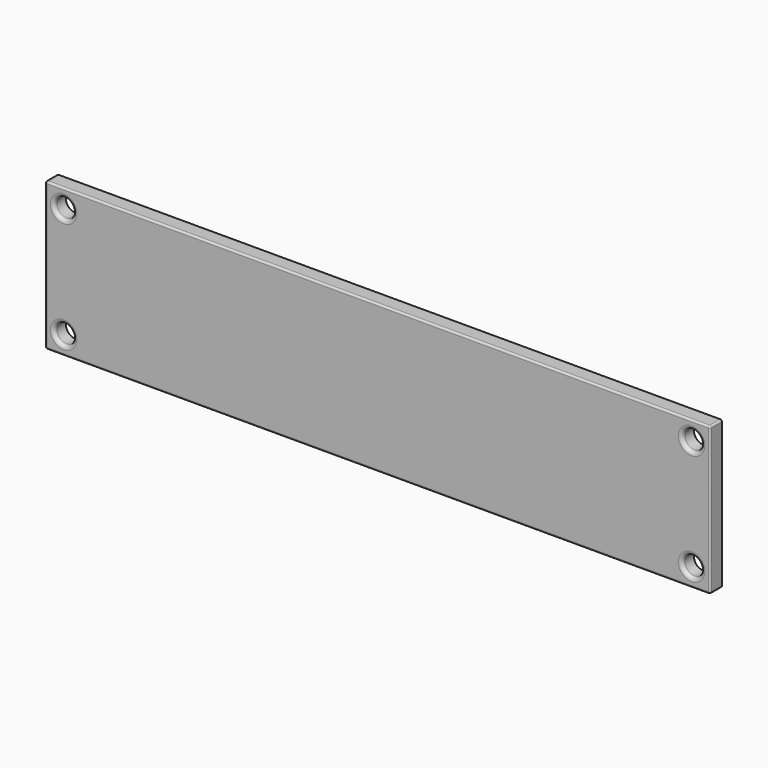
from build123d import *

# Parameters (mm, degrees)
F0_W         = 180
F0_H         = 40
F0_R         = 2.5751263091
F1_DEPTH     = 4
F2_R         = 1
F3_R         = 0.5
F4_TEXT_SIZE = 10.8600356345
F5_DEPTH     = 1


# Not quite as in the source:
# - a feature names something its author has since deleted; it is built from what else it names
# - Text() gives the source's letters only with a copy of the font that has no kerning and outlines rounded to 1/6400 em; it was checked with that copy


with BuildPart() as f1:
    # F0 (on Front) → F1 (new body)
    with BuildSketch(Plane.XZ):
        Rectangle(F0_W, F0_H)
        with Locations((-85, -15)):
            Circle(F0_R, mode=Mode.SUBTRACT)
        with Locations((85, -15)):
            Circle(F0_R, mode=Mode.SUBTRACT)
        with Locations((-85, 15)):
            Circle(F0_R, mode=Mode.SUBTRACT)
        with Locations((85, 15)):
            Circle(F0_R, mode=Mode.SUBTRACT)
    extrude(amount=F1_DEPTH)

    # F2
    f2_edges = [f1.edges().sort_by_distance(p)[0] for p in [
        (-87.575126, -4, 15),
        (-87.575126, -4, -15),
        (82.424874, -4, 15),
        (82.424874, -4, -15),
    ]]
    fillet(f2_edges, radius=F2_R)

    # F3
    f3_edges = [f1.edges().sort_by_distance(p)[0] for p in [
        (0, -4, 20),
        (-90, -4, 0),
        (0, -4, -20),
        (90, -4, 0),
        (-90, -2, 20),
        (-90, -2, -20),
        (90, -2, 20),
        (90, -2, -20),
    ]]
    fillet(f3_edges, radius=F3_R)

    # F4 (on face) → F5 (join)
    with BuildSketch(Plane(origin=(0, 0, 0), x_dir=(-1, 0, 0), z_dir=(0, 1, 0))):
        with Locations((-67.0410394669, 0)):
            Text('Havana Cap', F4_TEXT_SIZE, font='Open Sans', text_align=(TextAlign.LEFT, TextAlign.BOTTOM))
    extrude(amount=F5_DEPTH)

    # F6: F1 across plane


with BuildPart() as f1_1:
    add(f1.part)
    add(f1.part.mirror(Plane.YZ))


solid = f1_1.part
